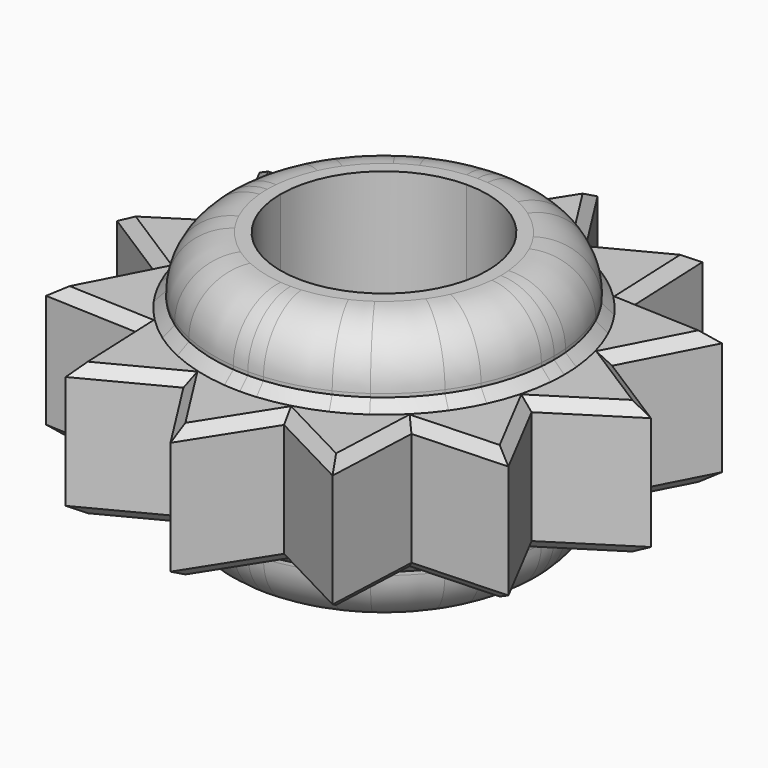
from build123d import *

# Parameters (mm, degrees)
F1_DEPTH      = 4
F2_DEPTH      = 6
F2_DEPTH_BACK = 2
F3_SIZE       = 0.3
F4_R          = 1.6
F5_SCALE      = 2


with BuildPart() as f1:
    # F0 (on Top) → F1 (new body)
    with BuildSketch(Plane.XY):
        with BuildLine():
            Line((8, 0), (5.1, 0))
            ThreePointArc((5.1, 0), (5.094966, -0.22655), (5.079873, -0.452653))
            Line((5.079873, -0.452653), (5.630053, -1.508568))
            Line((5.630053, -1.508568), (8, 0))
        make_face()
        with BuildLine():
            ThreePointArc((5.079873, 0.452653), (5.094966, 0.22655), (5.1, 0))
            Line((5.1, 0), (8, 0))
            Line((8, 0), (5.630053, 1.508568))
            Line((5.630053, 1.508568), (5.079873, 0.452653))
        make_face()
        with BuildLine():
            Line((0, 8), (0, 5.1))
            ThreePointArc((0, 5.1), (0.22655, 5.094966), (0.452653, 5.079873))
            Line((0.452653, 5.079873), (1.508568, 5.630053))
            Line((1.508568, 5.630053), (0, 8))
        make_face()
        with BuildLine():
            ThreePointArc((-0.452653, 5.079873), (-0.22655, 5.094966), (0, 5.1))
            Line((0, 5.1), (0, 8))
            Line((0, 8), (-1.508568, 5.630053))
            Line((-1.508568, 5.630053), (-0.452653, 5.079873))
        make_face()
        with BuildLine():
            Line((0, -8), (0, -5.1))
            ThreePointArc((0, -5.1), (-0.22655, -5.094966), (-0.452653, -5.079873))
            Line((-0.452653, -5.079873), (-1.508568, -5.630053))
            Line((-1.508568, -5.630053), (0, -8))
        make_face()
        with BuildLine():
            ThreePointArc((0.452653, -5.079873), (0.22655, -5.094966), (0, -5.1))
            Line((0, -5.1), (0, -8))
            Line((0, -8), (1.508568, -5.630053))
            Line((1.508568, -5.630053), (0.452653, -5.079873))
        make_face()
        with BuildLine():
            ThreePointArc((4.625625, 2.147928), (4.926222, 1.319977), (5.079873, 0.452653))
            Line((5.079873, 0.452653), (5.630053, 1.508568))
            Line((5.630053, 1.508568), (4.625625, 2.147928))
        make_face()
        with BuildLine():
            Line((5.630053, -1.508568), (5.079873, -0.452653))
            ThreePointArc((5.079873, -0.452653), (4.926222, -1.319977), (4.625625, -2.147928))
            Line((4.625625, -2.147928), (5.630053, -1.508568))
        make_face()
        with BuildLine():
            Line((-8, 0), (-5.1, 0))
            ThreePointArc((-5.1, 0), (-5.094966, 0.22655), (-5.079873, 0.452653))
            Line((-5.079873, 0.452653), (-5.630053, 1.508568))
            Line((-5.630053, 1.508568), (-8, 0))
        make_face()
        with BuildLine():
            ThreePointArc((-5.079873, -0.452653), (-5.094966, -0.22655), (-5.1, 0))
            Line((-5.1, 0), (-8, 0))
            Line((-8, 0), (-5.630053, -1.508568))
            Line((-5.630053, -1.508568), (-5.079873, -0.452653))
        make_face()
        with BuildLine():
            Line((1.508568, 5.630053), (0.452653, 5.079873))
            ThreePointArc((0.452653, 5.079873), (1.319977, 4.926222), (2.147928, 4.625625))
            Line((2.147928, 4.625625), (1.508568, 5.630053))
        make_face()
        with BuildLine():
            ThreePointArc((-2.147928, 4.625625), (-1.319977, 4.926222), (-0.452653, 5.079873))
            Line((-0.452653, 5.079873), (-1.508568, 5.630053))
            Line((-1.508568, 5.630053), (-2.147928, 4.625625))
        make_face()
        with BuildLine():
            Line((-1.508568, -5.630053), (-0.452653, -5.079873))
            ThreePointArc((-0.452653, -5.079873), (-1.319977, -4.926222), (-2.147928, -4.625625))
            Line((-2.147928, -4.625625), (-1.508568, -5.630053))
        make_face()
        with BuildLine():
            ThreePointArc((2.147928, -4.625625), (1.319977, -4.926222), (0.452653, -5.079873))
            Line((0.452653, -5.079873), (1.508568, -5.630053))
            Line((1.508568, -5.630053), (2.147928, -4.625625))
        make_face()
        with BuildLine():
            ThreePointArc((4.172972, 2.931945), (4.41673, 2.55), (4.625625, 2.147928))
            Line((4.625625, 2.147928), (5.630053, 1.508568))
            Line((5.630053, 1.508568), (6.928203, 4))
            Line((6.928203, 4), (4.121485, 4.121485))
            Line((4.121485, 4.121485), (4.172972, 2.931945))
        make_face()
        with BuildLine():
            Line((5.630053, -1.508568), (4.625625, -2.147928))
            ThreePointArc((4.625625, -2.147928), (4.41673, -2.55), (4.172972, -2.931945))
            Line((4.172972, -2.931945), (4.121485, -4.121485))
            Line((4.121485, -4.121485), (6.928203, -4))
            Line((6.928203, -4), (5.630053, -1.508568))
        make_face()
        with BuildLine():
            Line((-5.630053, 1.508568), (-5.079873, 0.452653))
            ThreePointArc((-5.079873, 0.452653), (-4.926222, 1.319977), (-4.625625, 2.147928))
            Line((-4.625625, 2.147928), (-5.630053, 1.508568))
        make_face()
        with BuildLine():
            ThreePointArc((-4.625625, -2.147928), (-4.926222, -1.319977), (-5.079873, -0.452653))
            Line((-5.079873, -0.452653), (-5.630053, -1.508568))
            Line((-5.630053, -1.508568), (-4.625625, -2.147928))
        make_face()
        with BuildLine():
            Line((1.508568, 5.630053), (2.147928, 4.625625))
            ThreePointArc((2.147928, 4.625625), (2.55, 4.41673), (2.931945, 4.172972))
            Line((2.931945, 4.172972), (4.121485, 4.121485))
            Line((4.121485, 4.121485), (4, 6.928203))
            Line((4, 6.928203), (1.508568, 5.630053))
        make_face()
        with BuildLine():
            ThreePointArc((-2.931945, 4.172972), (-2.55, 4.41673), (-2.147928, 4.625625))
            Line((-2.147928, 4.625625), (-1.508568, 5.630053))
            Line((-1.508568, 5.630053), (-4, 6.928203))
            Line((-4, 6.928203), (-4.121485, 4.121485))
            Line((-4.121485, 4.121485), (-2.931945, 4.172972))
        make_face()
        with BuildLine():
            Line((-1.508568, -5.630053), (-2.147928, -4.625625))
            ThreePointArc((-2.147928, -4.625625), (-2.55, -4.41673), (-2.931945, -4.172972))
            Line((-2.931945, -4.172972), (-4.121485, -4.121485))
            Line((-4.121485, -4.121485), (-4, -6.928203))
            Line((-4, -6.928203), (-1.508568, -5.630053))
        make_face()
        with BuildLine():
            ThreePointArc((2.931945, -4.172972), (2.55, -4.41673), (2.147928, -4.625625))
            Line((2.147928, -4.625625), (1.508568, -5.630053))
            Line((1.508568, -5.630053), (4, -6.928203))
            Line((4, -6.928203), (4.121485, -4.121485))
            Line((4.121485, -4.121485), (2.931945, -4.172972))
        make_face()
        with BuildLine():
            ThreePointArc((2.931945, 4.172972), (3.606245, 3.606245), (4.172972, 2.931945))
            Line((4.172972, 2.931945), (4.121485, 4.121485))
            Line((4.121485, 4.121485), (2.931945, 4.172972))
        make_face()
        with BuildLine():
            Line((4.121485, -4.121485), (4.172972, -2.931945))
            ThreePointArc((4.172972, -2.931945), (3.606245, -3.606245), (2.931945, -4.172972))
            Line((2.931945, -4.172972), (4.121485, -4.121485))
        make_face()
        with BuildLine():
            Line((-5.630053, 1.508568), (-4.625625, 2.147928))
            ThreePointArc((-4.625625, 2.147928), (-4.41673, 2.55), (-4.172972, 2.931945))
            Line((-4.172972, 2.931945), (-4.121485, 4.121485))
            Line((-4.121485, 4.121485), (-6.928203, 4))
            Line((-6.928203, 4), (-5.630053, 1.508568))
        make_face()
        with BuildLine():
            ThreePointArc((-4.172972, -2.931945), (-4.41673, -2.55), (-4.625625, -2.147928))
            Line((-4.625625, -2.147928), (-5.630053, -1.508568))
            Line((-5.630053, -1.508568), (-6.928203, -4))
            Line((-6.928203, -4), (-4.121485, -4.121485))
            Line((-4.121485, -4.121485), (-4.172972, -2.931945))
        make_face()
        with BuildLine():
            ThreePointArc((-4.172972, 2.931945), (-3.606245, 3.606245), (-2.931945, 4.172972))
            Line((-2.931945, 4.172972), (-4.121485, 4.121485))
            Line((-4.121485, 4.121485), (-4.172972, 2.931945))
        make_face()
        with BuildLine():
            Line((-4.121485, -4.121485), (-2.931945, -4.172972))
            ThreePointArc((-2.931945, -4.172972), (-3.606245, -3.606245), (-4.172972, -2.931945))
            Line((-4.172972, -2.931945), (-4.121485, -4.121485))
        make_face()
    extrude(amount=F1_DEPTH)

    # F0 (on Top) → F2 (join, two sides)
    with BuildSketch(Plane.XY) as f2_sk:
        with BuildLine():
            ThreePointArc((-3.1, 0), (-2.192031, 2.192031), (0, 3.1))
            Line((0, 3.1), (0, 5.1))
            ThreePointArc((0, 5.1), (-0.22655, 5.094966), (-0.452653, 5.079873))
            ThreePointArc((-0.452653, 5.079873), (-1.319977, 4.926222), (-2.147928, 4.625625))
            ThreePointArc((-2.147928, 4.625625), (-2.55, 4.41673), (-2.931945, 4.172972))
            ThreePointArc((-2.931945, 4.172972), (-3.606245, 3.606245), (-4.172972, 2.931945))
            ThreePointArc((-4.172972, 2.931945), (-4.41673, 2.55), (-4.625625, 2.147928))
            ThreePointArc((-4.625625, 2.147928), (-4.926222, 1.319977), (-5.079873, 0.452653))
            ThreePointArc((-5.079873, 0.452653), (-5.094966, 0.22655), (-5.1, 0))
            Line((-5.1, 0), (-3.1, 0))
        make_face()
        with BuildLine():
            ThreePointArc((0, 3.1), (2.192031, 2.192031), (3.1, 0))
            Line((3.1, 0), (5.1, 0))
            ThreePointArc((5.1, 0), (5.094966, 0.22655), (5.079873, 0.452653))
            ThreePointArc((5.079873, 0.452653), (4.926222, 1.319977), (4.625625, 2.147928))
            ThreePointArc((4.625625, 2.147928), (4.41673, 2.55), (4.172972, 2.931945))
            ThreePointArc((4.172972, 2.931945), (3.606245, 3.606245), (2.931945, 4.172972))
            ThreePointArc((2.931945, 4.172972), (2.55, 4.41673), (2.147928, 4.625625))
            ThreePointArc((2.147928, 4.625625), (1.319977, 4.926222), (0.452653, 5.079873))
            ThreePointArc((0.452653, 5.079873), (0.22655, 5.094966), (0, 5.1))
            Line((0, 5.1), (0, 3.1))
        make_face()
        with BuildLine():
            Line((0, -5.1), (0, -3.1))
            ThreePointArc((0, -3.1), (-2.192031, -2.192031), (-3.1, 0))
            Line((-3.1, 0), (-5.1, 0))
            ThreePointArc((-5.1, 0), (-5.094966, -0.22655), (-5.079873, -0.452653))
            ThreePointArc((-5.079873, -0.452653), (-4.926222, -1.319977), (-4.625625, -2.147928))
            ThreePointArc((-4.625625, -2.147928), (-4.41673, -2.55), (-4.172972, -2.931945))
            ThreePointArc((-4.172972, -2.931945), (-3.606245, -3.606245), (-2.931945, -4.172972))
            ThreePointArc((-2.931945, -4.172972), (-2.55, -4.41673), (-2.147928, -4.625625))
            ThreePointArc((-2.147928, -4.625625), (-1.319977, -4.926222), (-0.452653, -5.079873))
            ThreePointArc((-0.452653, -5.079873), (-0.22655, -5.094966), (0, -5.1))
        make_face()
        with BuildLine():
            Line((5.1, 0), (3.1, 0))
            ThreePointArc((3.1, 0), (2.192031, -2.192031), (0, -3.1))
            Line((0, -3.1), (0, -5.1))
            ThreePointArc((0, -5.1), (0.22655, -5.094966), (0.452653, -5.079873))
            ThreePointArc((0.452653, -5.079873), (1.319977, -4.926222), (2.147928, -4.625625))
            ThreePointArc((2.147928, -4.625625), (2.55, -4.41673), (2.931945, -4.172972))
            ThreePointArc((2.931945, -4.172972), (3.606245, -3.606245), (4.172972, -2.931945))
            ThreePointArc((4.172972, -2.931945), (4.41673, -2.55), (4.625625, -2.147928))
            ThreePointArc((4.625625, -2.147928), (4.926222, -1.319977), (5.079873, -0.452653))
            ThreePointArc((5.079873, -0.452653), (5.094966, -0.22655), (5.1, 0))
        make_face()
    extrude(amount=F2_DEPTH)
    extrude(f2_sk.sketch, amount=-F2_DEPTH_BACK)

    # F3
    f3_edges = [f1.edges().sort_by_distance(p)[0] for p in [
        (6.815027, -0.754284, 0),
        (6.815027, 0.754284, 0),
        (6.279128, 2.754284, 0),
        (5.524844, 4.060742, 0),
        (4.060742, 5.524844, 0),
        (2.754284, 6.279128, 0),
        (0.754284, 6.815027, 0),
        (-0.754284, 6.815027, 0),
        (-2.754284, 6.279128, 0),
        (-4.060742, 5.524844, 0),
        (-5.524844, 4.060742, 0),
        (-6.279128, 2.754284, 0),
        (-6.815027, 0.754284, 0),
        (-6.815027, -0.754284, 0),
        (-6.279128, -2.754284, 0),
        (-5.524844, -4.060742, 0),
        (-4.060742, -5.524844, 0),
        (-2.754284, -6.279128, 0),
        (-0.754284, -6.815027, 0),
        (0.754284, -6.815027, 0),
        (2.754284, -6.279128, 0),
        (4.060742, -5.524844, 0),
        (5.524844, -4.060742, 0),
        (6.279128, -2.754284, 0),
        (0, 5.1, 0),
        (6.815027, -0.754284, 4),
        (6.815027, 0.754284, 4),
        (6.279128, 2.754284, 4),
        (5.524844, 4.060742, 4),
        (4.060742, 5.524844, 4),
        (2.754284, 6.279128, 4),
        (0.754284, 6.815027, 4),
        (-0.754284, 6.815027, 4),
        (-2.754284, 6.279128, 4),
        (-4.060742, 5.524844, 4),
        (-5.524844, 4.060742, 4),
        (-6.279128, 2.754284, 4),
        (-6.815027, 0.754284, 4),
        (-6.815027, -0.754284, 4),
        (-6.279128, -2.754284, 4),
        (-5.524844, -4.060742, 4),
        (-4.060742, -5.524844, 4),
        (-2.754284, -6.279128, 4),
        (-0.754284, -6.815027, 4),
        (0.754284, -6.815027, 4),
        (2.754284, -6.279128, 4),
        (4.060742, -5.524844, 4),
        (5.524844, -4.060742, 4),
        (6.279128, -2.754284, 4),
        (0, 5.1, 4),
    ]]
    chamfer(f3_edges, length=F3_SIZE)

    # F4
    f4_edges = [f1.edges().sort_by_distance(p)[0] for p in [
        (0, 5.1, 6),
        (0, 5.1, -2),
    ]]
    fillet(f4_edges, radius=F4_R)


with BuildPart() as f1_1:
    # F5: moved
    add(f1.part.scale(F5_SCALE))


solid = f1_1.part
